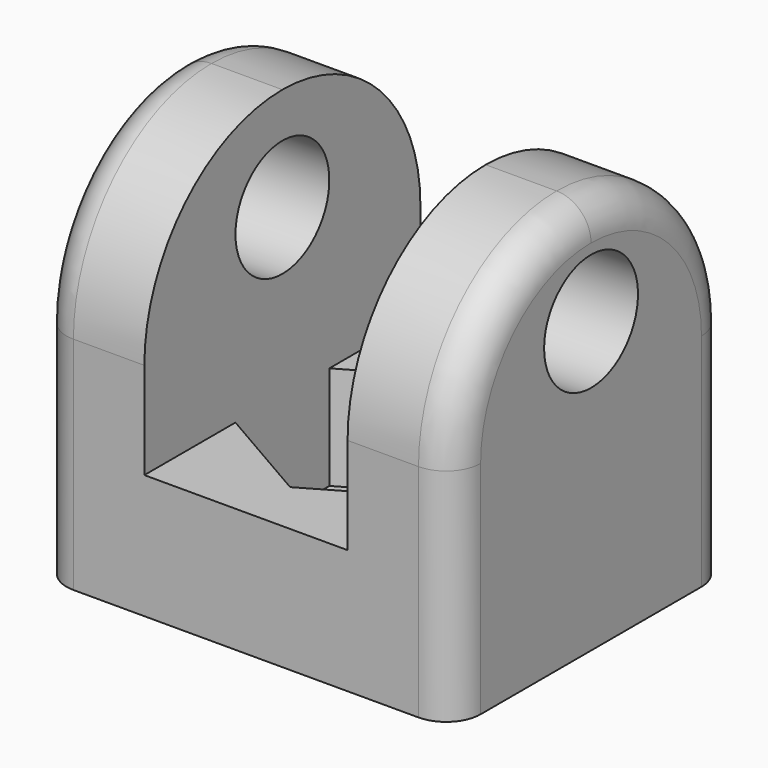
from build123d import *

# Parameters (mm, degrees)
F0_R     = 1.7
F5_DEPTH = 0.6
F6_DEPTH = 3.6
F7_DEPTH = 11.4
F8_D     = 3.4
F8_DEPTH = 5
F8_START = 1
F8_TIP   = 1.0214630523
F9_D     = 3.4
F9_DEPTH = 5
F9_START = 1
F9_TIP   = 1.0214630523
F10_R    = 4.99999
F11_R    = 1


# Not quite as in the source:
# - a fillet or chamfer is up to 0.001 mm smaller than in the source, because OpenCascade refuses the exact size


with BuildPart() as f5:
    # F0 (on Top) → F5 (new body)
    with BuildSketch(Plane.XY):
        Polygon((0, 3.4), (-2.9444863729, 1.7), (-2.9444863729, -1.7), (0, -3.4), (2.9444863729, -1.7), (2.9444863729, 1.7), align=None)
        Circle(F0_R, mode=Mode.SUBTRACT)
    extrude(amount=F5_DEPTH)

    # F0 (on Top) → F6 (join)
    with BuildSketch(Plane.XY):
        Polygon((2.9444863729, 5), (-2.9444863729, 5), (-2.9444863729, 1.7), (0, 3.4), (2.9444863729, 1.7), align=None)
        Polygon((-2.9444863729, -1.7), (-2.9444863729, -5), (2.9444863729, -5), (2.9444863729, -1.7), (0, -3.4), align=None)
    extrude(amount=F6_DEPTH)

    # F0 (on Top) → F7 (join)
    with BuildSketch(Plane.XY):
        Polygon((-2.9444863729, 5), (-6, 5), (-6, -5), (-2.9444863729, -5), (-2.9444863729, -1.7), (-2.9444863729, 1.7), align=None)
        Polygon((6, 5), (2.9444863729, 5), (2.9444863729, 1.7), (2.9444863729, -1.7), (2.9444863729, -5), (6, -5), align=None)
    extrude(amount=F7_DEPTH)

    # F8
    # its depths count from where the whole tool has entered the part; down to there all is cleared
    with Locations(Plane(origin=(-7, 0, 0), x_dir=(0, 1, 0), z_dir=(-1, 0, 0)).offset(-F8_START)):
        with Locations((0, -8.4)):
            Hole(F8_D / 2, depth=F8_DEPTH)
            with Locations((0, 0, -(F8_DEPTH + F8_TIP / 2))):  # 118° drill point
                Cone(0, F8_D / 2, F8_TIP, mode=Mode.SUBTRACT)

    # F9
    # its depths count from where the whole tool has entered the part; down to there all is cleared
    with Locations(Plane.YZ.offset(7).offset(-F9_START)):
        with Locations((0, 8.4)):
            Hole(F9_D / 2, depth=F9_DEPTH)
            with Locations((0, 0, -(F9_DEPTH + F9_TIP / 2))):  # 118° drill point
                Cone(0, F9_D / 2, F9_TIP, mode=Mode.SUBTRACT)

    # F10 (radius 5 in the source; OpenCascade refuses exactly that, so slightly less here)
    f10_edges = [f5.edges().sort_by_distance(p)[0] for p in [
        (-4.472243, -5, 11.4),
        (-4.472243, 5, 11.4),
        (4.472243, 5, 11.4),
        (4.472243, -5, 11.4),
    ]]
    fillet(f10_edges, radius=F10_R)

    # F11
    f11_edges = [f5.edges().sort_by_distance(p)[0] for p in [
        (6, 3.535537, 9.935537),
        (-6, 3.535537, 9.935537),
    ]]
    fillet(f11_edges, radius=F11_R)


solid = f5.part
